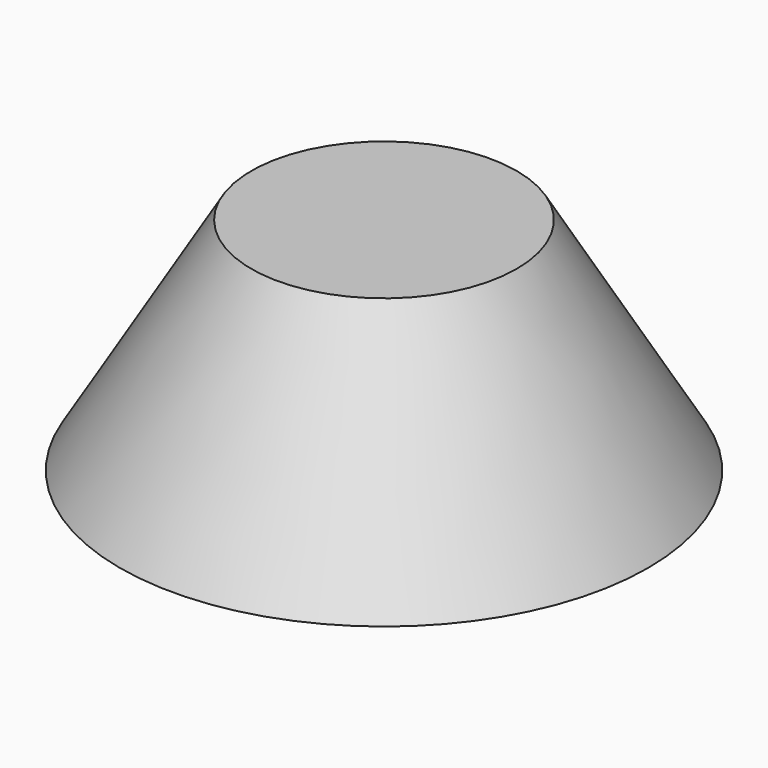
from build123d import *

# Parameters (mm, degrees)
F0_R = 45.6278244186
F2_R = 22.9267994929


with BuildPart() as f3:
    # F0 (on Top) → F3 section 0
    with BuildSketch(Plane.XY):
        Circle(F0_R)
    # F2 (on offset) → F3 section 1
    with BuildSketch(Plane.XY.offset(38.1)):
        Circle(F2_R)
    loft()


solid = f3.part
